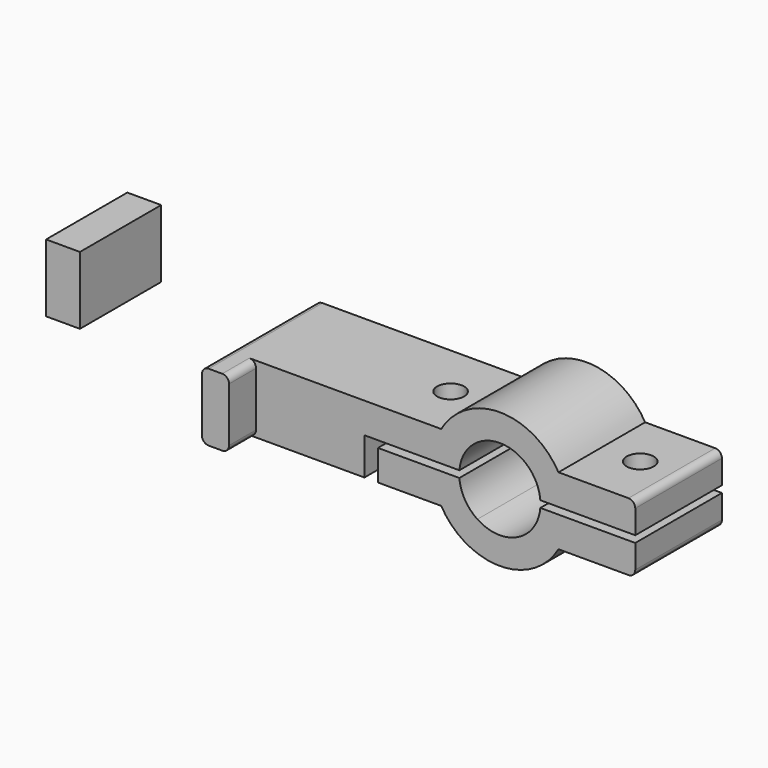
from build123d import *

# Parameters (mm, degrees)
F1_DEPTH  = 16
F2_W      = 4
F2_H      = 10
F3_DEPTH  = 5
F4_R      = 2
F5_DEPTH  = 25
F6_R      = 2
F7_DEPTH  = 3
F8_R      = 1
F8_2_R    = 1
F9_W      = 5
F9_H      = 15
F10_DEPTH = 10


with BuildPart() as f1:
    # F0 (on Front) → F1 (new body)
    with BuildSketch(Plane.XZ):
        with BuildLine():
            ThreePointArc((3.3166247904, 5), (5.1638421749, 3.0552796914), (5.9791303716, 0.5))
            Line((5.9791303716, 0.5), (9.9874921777, 0.5))
            ThreePointArc((9.9874921777, 0.5), (9.5915123797, 2.828938011), (8.6602540378, 5))
            Line((8.6602540378, 5), (3.3166247904, 5))
        make_face()
        with BuildLine():
            ThreePointArc((-3.3166247904, 5), (0, 6), (3.3166247904, 5))
            Line((3.3166247904, 5), (8.6602540378, 5))
            ThreePointArc((8.6602540378, 5), (0, 10), (-8.6602540378, 5))
            Line((-8.6602540378, 5), (-3.3166247904, 5))
        make_face()
        with BuildLine():
            ThreePointArc((8.6602540378, 5), (9.5915123797, 2.828938011), (9.9874921777, 0.5))
            Line((9.9874921777, 0.5), (20, 0.5))
            Line((20, 0.5), (20, 5))
            Line((20, 5), (8.6602540378, 5))
        make_face()
        with BuildLine():
            Line((-9.9874921777, 0.5), (-5.9791303716, 0.5))
            ThreePointArc((-5.9791303716, 0.5), (-5.1638421749, 3.0552796914), (-3.3166247904, 5))
            Line((-3.3166247904, 5), (-8.6602540378, 5))
            ThreePointArc((-8.6602540378, 5), (-9.5915123797, 2.828938011), (-9.9874921777, 0.5))
        make_face()
        with BuildLine():
            Line((-18, 0.5), (-9.9874921777, 0.5))
            ThreePointArc((-9.9874921777, 0.5), (-9.5915123797, 2.828938011), (-8.6602540378, 5))
            Line((-8.6602540378, 5), (-40, 5))
            Line((-40, 5), (-40, -5))
            Line((-40, -5), (-20, -5))
            Line((-20, -5), (-20, -0.5))
            Line((-20, -0.5), (-20, 0.5))
            Line((-20, 0.5), (-18, 0.5))
        make_face()
    extrude(amount=F1_DEPTH)

    # F2 (on face) → F3 (join)
    with BuildSketch(Plane.XZ.offset(16)):
        with Locations((-38, 0)):
            Rectangle(F2_W, F2_H)
    extrude(amount=F3_DEPTH)


with BuildPart() as f1b:
    # F0 (on Front) → F1, piece 2 (new body)
    with BuildSketch(Plane.XZ):
        with BuildLine():
            Line((9.9874921777, -0.5), (5.9791303716, -0.5))
            ThreePointArc((5.9791303716, -0.5), (5.1638421749, -3.0552796914), (3.3166247904, -5))
            Line((3.3166247904, -5), (8.6602540378, -5))
            ThreePointArc((8.6602540378, -5), (9.5915123797, -2.828938011), (9.9874921777, -0.5))
        make_face()
        with BuildLine():
            Line((8.6602540378, -5), (3.3166247904, -5))
            ThreePointArc((3.3166247904, -5), (0, -6), (-3.3166247904, -5))
            Line((-3.3166247904, -5), (-8.6602540378, -5))
            ThreePointArc((-8.6602540378, -5), (0, -10), (8.6602540378, -5))
        make_face()
        with BuildLine():
            Line((20, -0.5), (9.9874921777, -0.5))
            ThreePointArc((9.9874921777, -0.5), (9.5915123797, -2.828938011), (8.6602540378, -5))
            Line((8.6602540378, -5), (20, -5))
            Line((20, -5), (20, -0.5))
        make_face()
        with BuildLine():
            ThreePointArc((-3.3166247904, -5), (-5.1638421749, -3.0552796914), (-5.9791303716, -0.5))
            Line((-5.9791303716, -0.5), (-9.9874921777, -0.5))
            ThreePointArc((-9.9874921777, -0.5), (-9.5915123797, -2.828938011), (-8.6602540378, -5))
            Line((-8.6602540378, -5), (-3.3166247904, -5))
        make_face()
        with BuildLine():
            ThreePointArc((-8.6602540378, -5), (-9.5915123797, -2.828938011), (-9.9874921777, -0.5))
            Line((-9.9874921777, -0.5), (-18, -0.5))
            Line((-18, -0.5), (-18, -5))
            Line((-18, -5), (-8.6602540378, -5))
        make_face()
    extrude(amount=F1_DEPTH)


with BuildPart() as f5_tool:
    # F4 (on face) → F5 (new body)
    with BuildSketch(Plane(origin=(0, 0, -5), x_dir=(1, 0, 0), z_dir=(0, 0, -1))):
        with Locations((-13.6698729811, 8)):
            Circle(F4_R)
        with Locations((14.3301270189, 8)):
            Circle(F4_R)
    extrude(amount=-F5_DEPTH)


with BuildPart() as f1_1:
    add(f1.part)

    # F5: cut by f5_tool
    add(f5_tool.part, mode=Mode.SUBTRACT)

    # F8
    f8_edges = [f1_1.edges().sort_by_distance(p)[0] for p in [
        (20, -8, 5),
        (-40, -10.5, -5),
        (-40, -10.5, 5),
        (-36, -18.5, -5),
        (-36, -18.5, 5),
    ]]
    fillet(f8_edges, radius=F8_R)


with BuildPart() as f1b_1:
    add(f1b.part)

    # F5: cut by f5_tool
    add(f5_tool.part, mode=Mode.SUBTRACT)

    # F6 (on face) → F7 (cut)
    with BuildSketch(Plane(origin=(0, 0, -5), x_dir=(1, 0, 0), z_dir=(0, 0, -1))):
        Polygon((-15.4019237886, 5), (-11.9378221735, 5), (-10.2057713659, 8), (-11.9378221735, 11), (-15.4019237886, 11), (-17.1339745962, 8), align=None)
        with Locations((-13.6698729811, 8)):
            Circle(F6_R, mode=Mode.SUBTRACT)
        Polygon((12.5980762114, 5), (16.0621778265, 5), (17.7942286341, 8), (16.0621778265, 11), (12.5980762114, 11), (10.8660254038, 8), align=None)
        with Locations((14.3301270189, 8)):
            Circle(F6_R, mode=Mode.SUBTRACT)
    extrude(amount=-F7_DEPTH, mode=Mode.SUBTRACT)

    # F8#2
    f8_2_edges = [f1b_1.edges().sort_by_distance(p)[0] for p in [
        (20, -8, -5),
    ]]
    fillet(f8_2_edges, radius=F8_2_R)


with BuildPart() as f10:
    # F9 (on Top) → F10 (new body)
    with BuildSketch(Plane.XY):
        with Locations((-65.3190290928, -7.5)):
            Rectangle(F9_W, F9_H)
    extrude(amount=F10_DEPTH)


solid = Compound([f1_1.part, f1b_1.part, f10.part])
